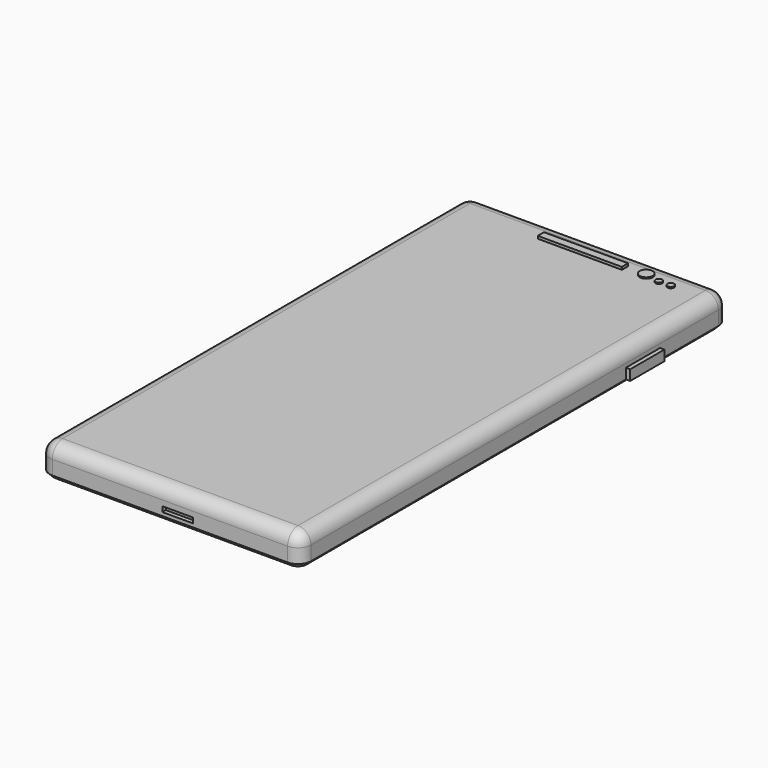
from build123d import *

# Parameters (mm, degrees)
F0_W          = 60.5537816882
F0_H          = 124.0280978382
F1_DEPTH      = 7.3
F2_R          = 3
F3_R          = 3
F4_R          = 3
F6_W          = 19.499885384
F6_H          = 1.8146336079
F7_DEPTH      = 0.3
F8_R          = 1.5145743504
F8_R_2        = 0.7515212849
F8_R_3        = 0.7715337707
F7_FACE_W     = 19.499885384
F7_FACE_H     = 1.8146336079
F9_DEPTH      = 0.3
F10_SIZE      = 1
F11_W         = 9.6169358585
F11_H         = 9.979840368
F12_DEPTH     = 1
F13_R         = 1
F14_SIZE      = 0.99999
F15_W         = 3.3568050712
F15_H         = 8.6971707642
F16_DEPTH     = 0.3
F17_W         = 3.7423321046
F17_H         = 9.4268880785
F18_DEPTH     = 0.3
F19_R         = 0.3
F20_W         = 9.9072623998
F20_H         = 2.3864916768
F21_DEPTH     = 1
F22_W         = 8.2636941224
F22_H         = 2.2905719709
F22_W_2       = 7.5511187315
F23_DEPTH     = 1
F24_TEXT_SIZE = 2.3192110045
F25_DEPTH     = 0.5
F26_W         = 2.200441435
F26_H         = 0.5388839636
F27_DEPTH     = 0.5
F28_W         = 7.1084705414
F28_H         = 1.2057768181
F29_DEPTH     = 1
F30_R         = 1.2386900344
F31_DEPTH     = 4


# Not quite as in the source:
# - a fillet or chamfer is up to 0.001 mm smaller than in the source, because OpenCascade refuses the exact size
# - Text() gives the source's letters only with a copy of the font that has no kerning and outlines rounded to 1/6400 em; it was checked with that copy


with BuildPart() as f1:
    # F0 (on Top) → F1 (new body)
    with BuildSketch(Plane.XY):
        with Locations((3.109715879, -1.1711586267)):
            Rectangle(F0_W, F0_H)
    extrude(amount=F1_DEPTH)

    # F2
    f2_edges = [f1.edges().sort_by_distance(p)[0] for p in [
        (-27.167175, -1.171159, 7.3),
        (33.386607, -1.171159, 7.3),
    ]]
    fillet(f2_edges, radius=F2_R)

    # F3
    f3_edges = [f1.edges().sort_by_distance(p)[0] for p in [
        (3.109716, 60.84289, 7.3),
    ]]
    fillet(f3_edges, radius=F3_R)

    # F4
    f4_edges = [f1.edges().sort_by_distance(p)[0] for p in [
        (3.109716, -63.185208, 7.3),
    ]]
    fillet(f4_edges, radius=F4_R)

    # F6 (on face) → F7 (join)
    with BuildSketch(Plane.XY.offset(7.3)):
        with Locations((3.804292297, 55.6030198932)):
            Rectangle(F6_W, F6_H)
    extrude(amount=F7_DEPTH)

    # F8 (on face) + F7_face (on face) → F9 (join)
    with BuildSketch(Plane.XY.offset(7.3)):
        with Locations((18.232608214, 55.8988526464)):
            Circle(F8_R)
        with Locations((21.8003224581, 55.1098957658)):
            Circle(F8_R_2)
        with Locations((24.5182905346, 55.1651753485)):
            Circle(F8_R_3)
    with BuildSketch(Plane(origin=(3.804292297, 55.6030198932, 7.6), x_dir=(1, 0, 0), z_dir=(0, 0, 1))):
        Rectangle(F7_FACE_W, F7_FACE_H)
    extrude(amount=F9_DEPTH)

    # F10
    f10_edges = [f1.edges().sort_by_distance(p)[0] for p in [
        (33.386607, -1.171159, 0),
        (3.109716, 60.84289, 0),
        (-27.167175, -1.171159, 0),
        (32.507927, -62.306528, 0),
        (32.507927, 59.964211, 0),
        (3.109716, -63.185208, 0),
        (-26.288495, -62.306528, 0),
        (-26.288495, 59.964211, 0),
    ]]
    chamfer(f10_edges, length=F10_SIZE)

    # F11 (on face) → F12 (join)
    with BuildSketch(Plane(origin=(0, 0, 0), x_dir=(1, 0, 0), z_dir=(0, 0, -1))):
        with Locations((1.4516127994, -35.7459690422)):
            Rectangle(F11_W, F11_H)
    extrude(amount=F12_DEPTH)

    # F13
    f13_edges = [f1.edges().sort_by_distance(p)[0] for p in [
        (-3.356855, 40.735889, -0.5),
        (-3.356855, 30.756049, -0.5),
        (6.260081, 30.756049, -0.5),
        (6.260081, 40.735889, -0.5),
    ]]
    fillet(f13_edges, radius=F13_R)

    # F14 (size 1 in the source; OpenCascade refuses exactly that, so slightly less here)
    f14_edges = [f1.edges().sort_by_distance(p)[0] for p in [
        (6.260081, 35.745969, -1),
    ]]
    chamfer(f14_edges, length=F14_SIZE)

    # F15 (on face) → F16 (join)
    with BuildSketch(Plane(origin=(0, 0, 0), x_dir=(1, 0, 0), z_dir=(0, 0, -1))):
        with Locations((10.4151125997, -35.8073208481)):
            Rectangle(F15_W, F15_H)
    extrude(amount=F16_DEPTH)

    # F17 (on face) → F18 (join)
    with BuildSketch(Plane(origin=(0, 0, 0), x_dir=(1, 0, 0), z_dir=(0, 0, -1))):
        with Locations((-8.3923588973, -35.8124766499)):
            Rectangle(F17_W, F17_H)
    extrude(amount=F18_DEPTH)

    # F19
    f19_edges = [f1.edges().sort_by_distance(p)[0] for p in [
        (-10.263525, 40.525921, -0.15),
        (-10.263525, 31.099033, -0.15),
        (-6.521193, 31.099033, -0.15),
        (-6.521193, 40.525921, -0.15),
    ]]
    fillet(f19_edges, radius=F19_R)

    # F20 (on face) → F21 (join)
    with BuildSketch(Plane.YZ.offset(33.3866067231)):
        with Locations((36.0090760514, 2.1932458384)):
            Rectangle(F20_W, F20_H)
    extrude(amount=F21_DEPTH)

    # F22 (on face) → F23 (join)
    with BuildSketch(Plane(origin=(-27.1671749651, 0, 0), x_dir=(0, -1, 0), z_dir=(-1, 0, 0))):
        with Locations((-34.0711725876, 2.1452859854)):
            Rectangle(F22_W, F22_H)
        with Locations((-22.2886223346, 2.1452859854)):
            Rectangle(F22_W_2, F22_H)
    extrude(amount=F23_DEPTH)

    # F24 (on face) → F25 (cut)
    with BuildSketch(Plane(origin=(-28.1671749651, 0, 0), x_dir=(0, -1, 0), z_dir=(-1, 0, 0))):
        with Locations((-34.8540171981, 1.3349872315)):
            Text('+', F24_TEXT_SIZE, font='Open Sans', text_align=(TextAlign.LEFT, TextAlign.BOTTOM))
    extrude(amount=-F25_DEPTH, mode=Mode.SUBTRACT)

    # F26 (on face) → F27 (cut)
    with BuildSketch(Plane(origin=(-28.1671749651, 0, 0), x_dir=(0, -1, 0), z_dir=(-1, 0, 0))):
        with Locations((-22.1025450155, 2.1007956238)):
            Rectangle(F26_W, F26_H)
    extrude(amount=-F27_DEPTH, mode=Mode.SUBTRACT)

    # F28 (on face) → F29 (cut)
    with BuildSketch(Plane.XZ.offset(63.1852075458)):
        with Locations((4.9134622677, 2.4241241626)):
            Rectangle(F28_W, F28_H)
    extrude(amount=-F29_DEPTH, mode=Mode.SUBTRACT)

    # F30 (on face) → F31 (cut)
    with BuildSketch(Plane(origin=(0, 60.8428902924, 0), x_dir=(-1, 0, 0), z_dir=(0, 1, 0))):
        with Locations((16.2681862712, 2.5970449205)):
            Circle(F30_R)
    extrude(amount=-F31_DEPTH, mode=Mode.SUBTRACT)


solid = f1.part
